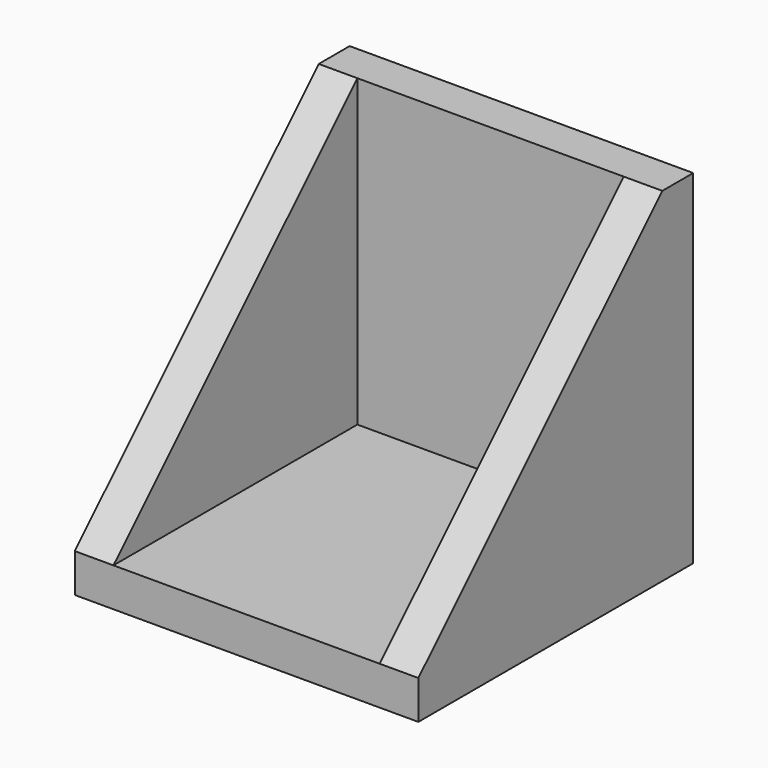
from build123d import *

# Parameters (mm, degrees)
F0_W     = 40
F0_H     = 40
F1_DEPTH = 40
F2_T     = -4.5
F3_SIZE  = 35.5


with BuildPart() as f1:
    # F0 (on Top) → F1 (new body)
    with BuildSketch(Plane.XY):
        Rectangle(F0_W, F0_H)
    extrude(amount=F1_DEPTH)

    # F2
    f2_openings = [f1.faces().sort_by_distance(p)[0] for p in [
        (0, -20, 20),
        (0, 0, 40),
    ]]
    offset(amount=F2_T, openings=f2_openings)

    # F3
    f3_edges = [f1.edges().sort_by_distance(p)[0] for p in [
        (-17.75, -20, 40),
        (17.75, -20, 40),
    ]]
    chamfer(f3_edges, length=F3_SIZE)


solid = f1.part
